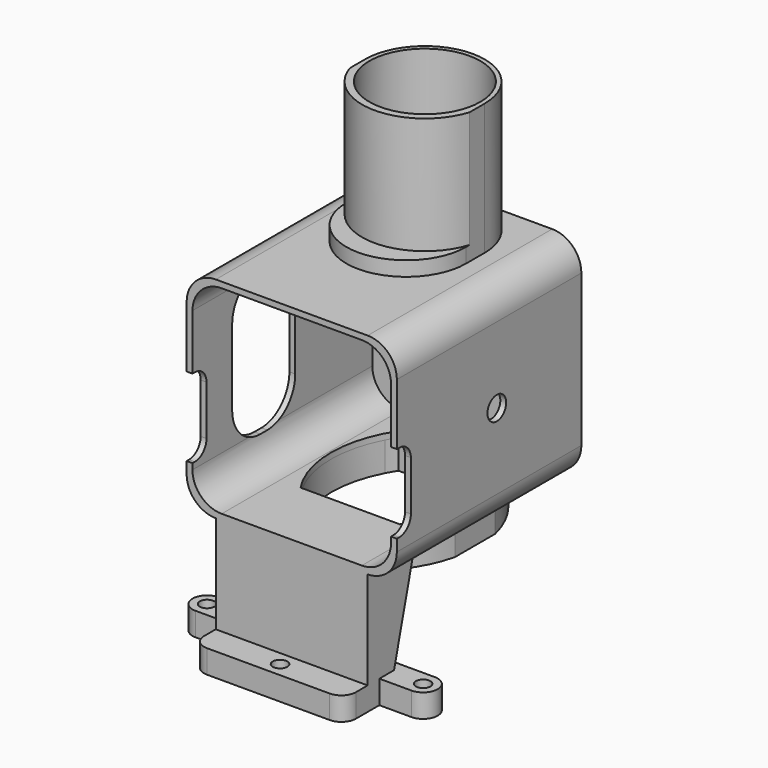
from build123d import *

# Parameters (mm, degrees)
F0_R      = 11.5
F1_DEPTH  = 2
F3_DEPTH  = 77
F5_DEPTH  = 3
F7_DEPTH  = 3
F9_DEPTH  = 5
F11_DEPTH = 3
F12_R     = 19
F13_DEPTH = 8
F14_R     = 19
F15_DEPTH = 40
F16_W     = 52
F16_H     = 3
F17_DEPTH = 38.5
F19_DEPTH = 3
F21_DEPTH = 10
F22_W     = 3
F22_H     = 38.5
F23_DEPTH = 5
F25_R     = 2.5
F25_W     = 47
F25_H     = 2
F26_DEPTH = 5
F27_DEPTH = 1
F29_DEPTH = 75
F30_DEPTH = 2
F24_W     = 3
F24_H     = 38.5
F31_DEPTH = 5
F32_R     = 4
F33_DEPTH = 3


with BuildPart() as f1:
    # F0 (on Front) → F1 (new body)
    with BuildSketch(Plane.XZ):
        with BuildLine():
            Line((26, 36), (-26, 36))
            ThreePointArc((-26, 36), (-33.0710678119, 33.0710678119), (-36, 26))
            Line((-36, 26), (-36, -26))
            ThreePointArc((-36, -26), (-33.0710678119, -33.0710678119), (-26, -36))
            Line((-26, -36), (26, -36))
            ThreePointArc((26, -36), (33.0710678119, -33.0710678119), (36, -26))
            Line((36, -26), (36, 26))
            ThreePointArc((36, 26), (33.0710678119, 33.0710678119), (26, 36))
        make_face()
        with BuildLine():
            Line((24, -34), (-24, -34))
            ThreePointArc((-24, -34), (-31.0710678119, -31.0710678119), (-34, -24))
            Line((-34, -24), (-34, 24))
            ThreePointArc((-34, 24), (-31.0710678119, 31.0710678119), (-24, 34))
            Line((-24, 34), (24, 34))
            ThreePointArc((24, 34), (31.0710678119, 31.0710678119), (34, 24))
            Line((34, 24), (34, -24))
            ThreePointArc((34, -24), (31.0710678119, -31.0710678119), (24, -34))
        make_face(mode=Mode.SUBTRACT)
        with BuildLine():
            ThreePointArc((-34, -24), (-31.0710678119, -31.0710678119), (-24, -34))
            Line((-24, -34), (24, -34))
            ThreePointArc((24, -34), (31.0710678119, -31.0710678119), (34, -24))
            Line((34, -24), (34, 24))
            ThreePointArc((34, 24), (31.0710678119, 31.0710678119), (24, 34))
            Line((24, 34), (-24, 34))
            ThreePointArc((-24, 34), (-31.0710678119, 31.0710678119), (-34, 24))
            Line((-34, 24), (-34, -24))
        make_face()
        Circle(F0_R, mode=Mode.SUBTRACT)
    extrude(amount=F1_DEPTH)

    # F2 (on face) → F3 (join)
    with BuildSketch(Plane.XZ.offset(2)):
        with BuildLine():
            Line((26, 36), (-26, 36))
            ThreePointArc((-26, 36), (-33.0710678119, 33.0710678119), (-36, 26))
            Line((-36, 26), (-36, -26))
            ThreePointArc((-36, -26), (-33.0710678119, -33.0710678119), (-26, -36))
            Line((-26, -36), (26, -36))
            ThreePointArc((26, -36), (33.0710678119, -33.0710678119), (36, -26))
            Line((36, -26), (36, 26))
            ThreePointArc((36, 26), (33.0710678119, 33.0710678119), (26, 36))
        make_face()
        with BuildLine():
            Line((24, -34), (-24, -34))
            ThreePointArc((-24, -34), (-31.0710678119, -31.0710678119), (-34, -24))
            Line((-34, -24), (-34, 24))
            ThreePointArc((-34, 24), (-31.0710678119, 31.0710678119), (-24, 34))
            Line((-24, 34), (24, 34))
            ThreePointArc((24, 34), (31.0710678119, 31.0710678119), (34, 24))
            Line((34, 24), (34, -24))
            ThreePointArc((34, -24), (31.0710678119, -31.0710678119), (24, -34))
        make_face(mode=Mode.SUBTRACT)
    extrude(amount=F3_DEPTH)

    # F4 (on face) → F5 (cut)
    with BuildSketch(Plane(origin=(-36, 0, 0), x_dir=(0, -1, 0), z_dir=(-1, 0, 0))):
        with BuildLine():
            ThreePointArc((62, 13), (58.4852813742, 21.4852813742), (50, 25))
            Line((50, 25), (47, 25))
            ThreePointArc((47, 25), (38.5147186258, 21.4852813742), (35, 13))
            Line((35, 13), (35, -13))
            ThreePointArc((35, -13), (38.5147186258, -21.4852813742), (47, -25))
            Line((47, -25), (50, -25))
            ThreePointArc((50, -25), (58.4852813742, -21.4852813742), (62, -13))
            Line((62, -13), (62, 13))
        make_face()
    extrude(amount=-F5_DEPTH, mode=Mode.SUBTRACT)

    # F6 (on face) → F7 (cut)
    with BuildSketch(Plane.XY.offset(36)):
        with BuildLine():
            Line((19, -30), (19, -22))
            ThreePointArc((19, -22), (0, -3), (-19, -22))
            Line((-19, -22), (-19, -30))
            ThreePointArc((-19, -30), (0, -49), (19, -30))
        make_face()
    extrude(amount=-F7_DEPTH, mode=Mode.SUBTRACT)

    # F8 (on face) → F9 (join)
    with BuildSketch(Plane.XY.offset(36)):
        with BuildLine():
            Line((-20.5, -22), (-20.5, -30))
            ThreePointArc((-20.5, -30), (0, -50.5), (20.5, -30))
            Line((20.5, -30), (20.5, -22))
            ThreePointArc((20.5, -22), (0, -1.5), (-20.5, -22))
        make_face()
        with BuildLine():
            ThreePointArc((-19, -22), (0, -3), (19, -22))
            Line((19, -22), (19, -22.3025978408))
            Line((19, -22.3025978408), (19, -29.6974021592))
            Line((19, -29.6974021592), (19, -30))
            ThreePointArc((19, -30), (0, -49), (-19, -30))
            Line((-19, -30), (-19, -22))
        make_face(mode=Mode.SUBTRACT)
        with BuildLine():
            Line((19, -22.3025978408), (19, -22))
            ThreePointArc((19, -22), (0, -3), (-19, -22))
            Line((-19, -22), (-19, -30))
            ThreePointArc((-19, -30), (0, -49), (19, -30))
            Line((19, -30), (19, -29.6974021592))
            Line((19, -29.6974021592), (19, -22.3025978408))
        make_face()
    extrude(amount=F9_DEPTH)

    # F10 (on face) → F11 (join)
    with BuildSketch(Plane.XY.offset(36)):
        with BuildLine():
            Line((20.5, -30), (20.5, -22))
            ThreePointArc((20.5, -22), (0, -1.5), (-20.5, -22))
            Line((-20.5, -22), (-20.5, -30))
            ThreePointArc((-20.5, -30), (0, -50.5), (20.5, -30))
        make_face()
    extrude(amount=F11_DEPTH)

    # F12 (on face) → F13 (cut)
    with BuildSketch(Plane.XY.offset(41)):
        with Locations((0, -22)):
            Circle(F12_R)
    extrude(amount=-F13_DEPTH, mode=Mode.SUBTRACT)

    # F14 (on face) → F15 (join)
    with BuildSketch(Plane.XY.offset(41)):
        with BuildLine():
            Line((-20.5, -22), (-20.5, -28.4807406984))
            ThreePointArc((-20.5, -28.4807406984), (0, -43.5), (20.5, -28.4807406984))
            Line((20.5, -28.4807406984), (20.5, -22))
            ThreePointArc((20.5, -22), (0, -1.5), (-20.5, -22))
        make_face()
        with Locations((0, -22)):
            Circle(F14_R, mode=Mode.SUBTRACT)
    extrude(amount=F15_DEPTH)

    # F16 (on face) → F17 (join)
    with BuildSketch(Plane(origin=(0, 0, -36), x_dir=(1, 0, 0), z_dir=(0, 0, -1))):
        with Locations((0, 77.5)):
            Rectangle(F16_W, F16_H)
    extrude(amount=F17_DEPTH)

    # F18 (on face) → F19 (cut)
    with BuildSketch(Plane(origin=(0, 0, -36), x_dir=(1, 0, 0), z_dir=(0, 0, -1))):
        with BuildLine():
            Line((-17, 12), (17, 12))
            ThreePointArc((17, 12), (23.3298247558, 33), (17, 54))
            Line((17, 54), (-17, 54))
            ThreePointArc((-17, 54), (-23.3298247558, 33), (-17, 12))
        make_face()
    extrude(amount=-F19_DEPTH, mode=Mode.SUBTRACT)

    # F20 (on face) → F21 (join)
    with BuildSketch(Plane(origin=(0, 0, -36), x_dir=(1, 0, 0), z_dir=(0, 0, -1))):
        with BuildLine():
            ThreePointArc((19, 50.6158820109), (23.3298247558, 33), (19, 15.3841179891))
            Line((19, 15.3841179891), (19, 10))
            ThreePointArc((19, 10), (23.2866263695, 16.8090036252), (26, 24.3836521016))
            Line((26, 24.3836521016), (26, 41.6163478984))
            ThreePointArc((26, 41.6163478984), (23.2866263695, 49.1909963748), (19, 56))
            Line((19, 56), (19, 50.6158820109))
        make_face()
        with BuildLine():
            Line((-19, 56), (-19, 50.6158820109))
            ThreePointArc((-19, 50.6158820109), (-18.0437883513, 52.3338197434), (-17, 54))
            Line((-17, 54), (17, 54))
            ThreePointArc((17, 54), (18.0437883513, 52.3338197434), (19, 50.6158820109))
            Line((19, 50.6158820109), (19, 56))
            Line((19, 56), (-19, 56))
        make_face()
        with BuildLine():
            Line((-19, 10), (-19, 15.3841179891))
            ThreePointArc((-19, 15.3841179891), (-23.3298247558, 33), (-19, 50.6158820109))
            Line((-19, 50.6158820109), (-19, 56))
            ThreePointArc((-19, 56), (-23.2866263695, 49.1909963748), (-26, 41.6163478984))
            Line((-26, 41.6163478984), (-26, 24.3836521016))
            ThreePointArc((-26, 24.3836521016), (-23.2866263695, 16.8090036252), (-19, 10))
        make_face()
        with BuildLine():
            Line((17, 12), (-17, 12))
            ThreePointArc((-17, 12), (-18.0437883513, 13.6661802566), (-19, 15.3841179891))
            Line((-19, 15.3841179891), (-19, 10))
            Line((-19, 10), (19, 10))
            Line((19, 10), (19, 15.3841179891))
            ThreePointArc((19, 15.3841179891), (18.0437883513, 13.6661802566), (17, 12))
        make_face()
    extrude(amount=F21_DEPTH)

    # F22 (on face) → F23 (join)
    with BuildSketch(Plane.YZ.offset(26)):
        Polygon((-76, -36), (-76, -74.5), (-69, -74.5), (-59, -36), align=None)
        with Locations((-77.5, -55.25)):
            Rectangle(F22_W, F22_H)
    extrude(amount=-F23_DEPTH)

    # F25 (on face) → F26 (join)
    with BuildSketch(Plane(origin=(0, 0, -74.5), x_dir=(1, 0, 0), z_dir=(0, 0, -1))):
        with BuildLine():
            Line((37, 74), (26, 74))
            Line((26, 74), (21, 74))
            Line((21, 74), (-26, 74))
            Line((-26, 74), (-37, 74))
            ThreePointArc((-37, 74), (-42, 69), (-37, 64))
            Line((-37, 64), (37, 64))
            ThreePointArc((37, 64), (42, 69), (37, 74))
        make_face()
        with Locations((-37, 69)):
            Circle(F25_R, mode=Mode.SUBTRACT)
        with Locations((0, 69)):
            Circle(F25_R, mode=Mode.SUBTRACT)
        with Locations((37, 69)):
            Circle(F25_R, mode=Mode.SUBTRACT)
        Polygon((26, 79), (-26, 79), (-26, 76), (21, 76), (21, 74), (26, 74), align=None)
        with Locations((-2.5, 75)):
            Rectangle(F25_W, F25_H)
        with BuildLine():
            Line((-26.0336585343, 79), (-26, 79))
            Line((-26, 79), (26, 79))
            Line((26, 79), (26, 84))
            ThreePointArc((26, 84), (24.5355339059, 87.5355339059), (21, 89))
            Line((21, 89), (-21.0336585343, 89))
            ThreePointArc((-21.0336585343, 89), (-24.5691924402, 87.5355339059), (-26.0336585343, 84))
            Line((-26.0336585343, 84), (-26.0336585343, 79))
        make_face()
        with Locations((0, 84)):
            Circle(F25_R, mode=Mode.SUBTRACT)
    extrude(amount=-F26_DEPTH)

    # F27 (add): faces of the model
    f27_faces = [f1.faces().sort_by_distance(p)[0] for p in [
        (23.5, -77.5, -74.5),
        (-2.5, -77.5, -74.5),
        (23.5, -72.5, -74.5),
        (-26.0168292671, -79.5298586246, -74.5),
        (-41.1514718626, -69, -74.5),
    ]]
    extrude(f27_faces, amount=F27_DEPTH)

    # F28 (on face) → F29 (cut)
    with BuildSketch(Plane.YZ.offset(36)):
        with BuildLine():
            Line((-78, 5), (-79, 5))
            Line((-79, 5), (-79, -22))
            Line((-79, -22), (-78, -22))
            ThreePointArc((-78, -22), (-74.4644660941, -20.5355339059), (-73, -17))
            Line((-73, -17), (-73, 0))
            ThreePointArc((-73, 0), (-74.4644660941, 3.5355339059), (-78, 5))
        make_face()
    extrude(amount=-F29_DEPTH, mode=Mode.SUBTRACT)

    # F30 (add): a face of the model
    f30_faces = [f1.faces().sort_by_distance(p)[0] for p in [
        (-0.0056811519, -75.1326620312, -75.5),
    ]]
    extrude(f30_faces, amount=F30_DEPTH)

    # F24 (on face) → F31 (join)
    with BuildSketch(Plane(origin=(-26, 0, 0), x_dir=(0, -1, 0), z_dir=(-1, 0, 0))):
        with Locations((77.5, -55.25)):
            Rectangle(F24_W, F24_H)
        Polygon((69, -74.5), (76, -74.5), (76, -36), (59, -36), align=None)
    extrude(amount=-F31_DEPTH)

    # F32 (on face) → F33 (cut)
    with BuildSketch(Plane.YZ.offset(36)):
        with Locations((-36.2, 0)):
            Circle(F32_R)
    extrude(amount=-F33_DEPTH, mode=Mode.SUBTRACT)


solid = f1.part
